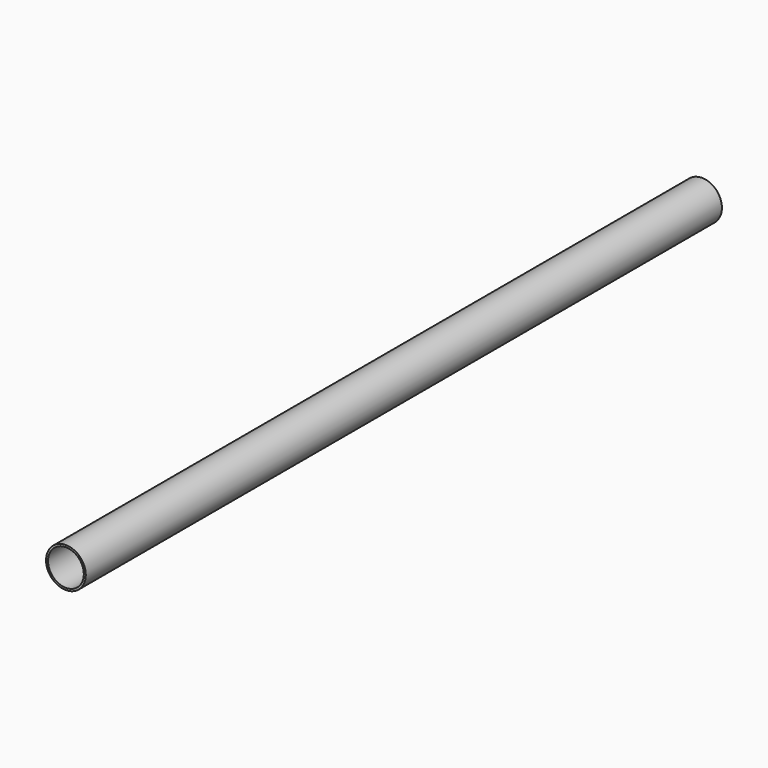
from build123d import *

# Parameters (mm, degrees)
F0_R     = 5
F0_R_2   = 4.5
F1_DEPTH = 120


# Not quite as in the source:
# - a pattern or mirror of a feature is missing from the dataset's text; its kind, count and spacing are read off the source's solid


with BuildPart() as f1:
    # F0 (on Front) → F1 (new body)
    with BuildSketch(Plane.XZ):
        Circle(F0_R)
        Circle(F0_R_2, mode=Mode.SUBTRACT)
    extrude(amount=F1_DEPTH)

    # F1_copies: F1 across plane


with BuildPart() as f1_1:
    add(f1.part)
    add(f1.part.mirror(Plane(origin=(0, -100, 0), x_dir=(0, 0, -1), z_dir=(0, -1, 0))))


solid = f1_1.part
